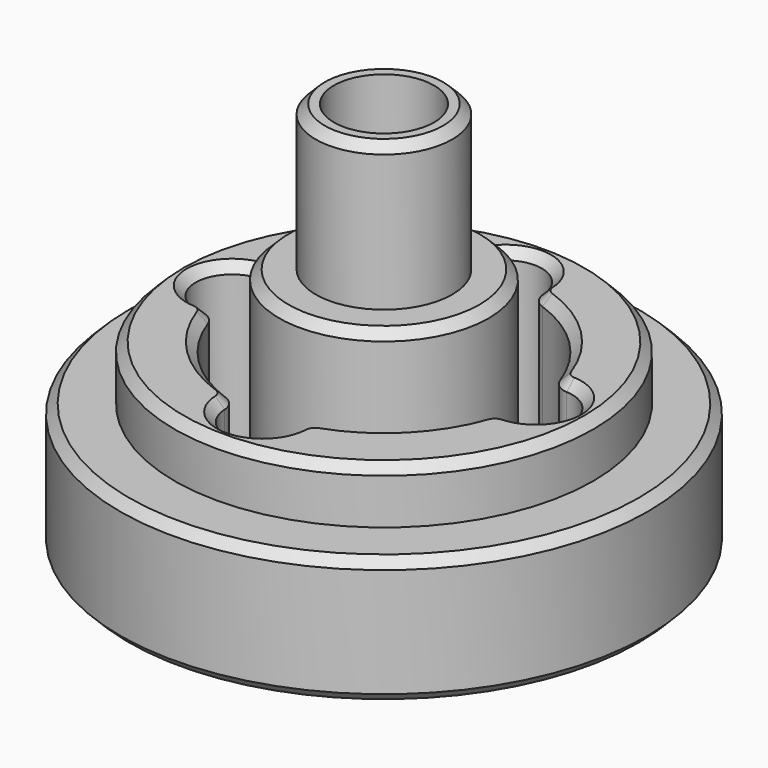
from build123d import *

# Parameters (mm, degrees)
F0_R      = 14.5
F1_DEPTH  = 10
F2_R      = 11.5
F3_DEPTH  = 9
F4_R      = 14.5
F4_R_2    = 11.5
F5_DEPTH  = 6
F6_R      = 25
F7_DEPTH  = 9
F8_R      = 1
F9_R      = 5.75
F10_DEPTH = 12.5
F11_R     = 3.75
F12_DEPTH = 8
F13_SIZE  = 0.5
F14_R     = 2.75
F15_DEPTH = 19


with BuildPart() as f1:
    # F0 (on Top) → F1 (new body)
    with BuildSketch(Plane.XY):
        Circle(F0_R)
    extrude(amount=F1_DEPTH)

    # F2 (on face) → F3 (join)
    with BuildSketch(Plane.XY.offset(10)):
        Circle(F2_R)
        with BuildLine():
            ThreePointArc((2, 7.7459666924), (5.6568542495, 5.6568542495), (7.7459666924, 2))
            Line((7.7459666924, 2), (8.3459666924, 2))
            ThreePointArc((8.3459666924, 2), (10.3459666924, 0), (8.3459666924, -2))
            Line((8.3459666924, -2), (7.7459666924, -2))
            ThreePointArc((7.7459666924, -2), (5.6568542495, -5.6568542495), (2, -7.7459666924))
            Line((2, -7.7459666924), (2, -8.3459666924))
            ThreePointArc((2, -8.3459666924), (0, -10.3459666924), (-2, -8.3459666924))
            Line((-2, -8.3459666924), (-2, -7.7459666924))
            ThreePointArc((-2, -7.7459666924), (-5.6568542495, -5.6568542495), (-7.7459666924, -2))
            Line((-7.7459666924, -2), (-8.3459666924, -2))
            ThreePointArc((-8.3459666924, -2), (-10.3459666924, 0), (-8.3459666924, 2))
            Line((-8.3459666924, 2), (-7.7459666924, 2))
            ThreePointArc((-7.7459666924, 2), (-5.6568542495, 5.6568542495), (-2, 7.7459666924))
            Line((-2, 7.7459666924), (-2, 8.3459666924))
            ThreePointArc((-2, 8.3459666924), (0, 10.3459666924), (2, 8.3459666924))
            Line((2, 8.3459666924), (2, 7.7459666924))
        make_face(mode=Mode.SUBTRACT)
    extrude(amount=F3_DEPTH)

    # F4 (on face) → F5 (join)
    with BuildSketch(Plane.XY.offset(10)):
        Circle(F4_R)
        Circle(F4_R_2, mode=Mode.SUBTRACT)
    extrude(amount=F5_DEPTH)

    # F6 (on face) → F7 (cut)
    with BuildSketch(Plane(origin=(0, 0, 0), x_dir=(1, 0, 0), z_dir=(0, 0, -1))):
        Circle(F6_R)
    extrude(amount=-F7_DEPTH, mode=Mode.SUBTRACT)

    # F8
    f8_edges = [f1.edges().sort_by_distance(p)[0] for p in [
        (-7.745967, 2, 14.5),
        (-2, 7.745967, 14.5),
        (2, 7.745967, 14.5),
        (7.745967, 2, 14.5),
        (-7.745967, -2, 14.5),
        (7.745967, -2, 14.5),
        (2, -7.745967, 14.5),
        (-2, -7.745967, 14.5),
    ]]
    fillet(f8_edges, radius=F8_R)

    # F9 (on face) → F10 (join)
    with BuildSketch(Plane.XY.offset(10)):
        Circle(F9_R)
    extrude(amount=F10_DEPTH)

    # F11 (on face) → F12 (join)
    with BuildSketch(Plane.XY.offset(22.5)):
        Circle(F11_R)
    extrude(amount=F12_DEPTH)

    # F13
    f13_edges = [f1.edges().sort_by_distance(p)[0] for p in [
        (-10.345967, 0, 19),
        (-7.889975, -2.194073, 19),
        (-7.889975, 2.194073, 19),
        (-5.656854, -5.656854, 19),
        (-5.656854, 5.656854, 19),
        (-2.194073, -7.889975, 19),
        (-2.194073, 7.889975, 19),
        (0, -10.345967, 19),
        (0, 10.345967, 19),
        (2.194073, -7.889975, 19),
        (2.194073, 7.889975, 19),
        (5.656854, -5.656854, 19),
        (5.656854, 5.656854, 19),
        (7.889975, -2.194073, 19),
        (7.889975, 2.194073, 19),
        (10.345967, 0, 19),
        (-11.5, 0, 19),
        (-14.5, 0, 16),
        (-3.75, 0, 30.5),
        (-5.75, 0, 22.5),
        (-14.5, 0, 9),
    ]]
    chamfer(f13_edges, length=F13_SIZE)

    # F14 (on face) → F15 (cut)
    with BuildSketch(Plane.XY.offset(30.5)):
        Circle(F14_R)
    extrude(amount=-F15_DEPTH, mode=Mode.SUBTRACT)


solid = f1.part
